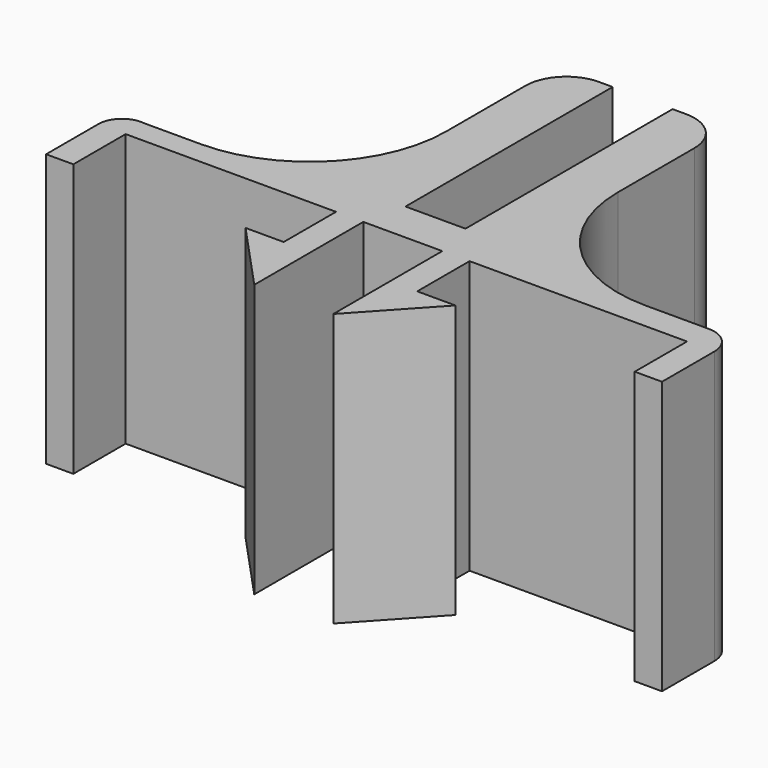
from build123d import *

# Parameters (mm, degrees)
F0_W     = 1
F0_H     = 2.4
F1_DEPTH = 10


# Not quite as in the source:
# - a feature names something its author has since deleted; it is built from what else it names


with BuildPart() as f1:
    # F0 (on Top) → F1 (new body)
    with BuildSketch(Plane.XY):
        with Locations((10.9311291858, -6.7)):
            Rectangle(F0_W, F0_H)
        with Locations((-10.6688708142, -6.7)):
            Rectangle(F0_W, F0_H)
        Polygon((-2.45, -8.5), (-2.45, -7.9), (-3.85, -7.9), (-1.45, -10.5), (-1.45, -8.5), align=None)
        with BuildLine():
            Line((-11.1688708142, -5.5), (-10.1688708142, -5.5))
            Line((-10.1688708142, -5.5), (-10.1688708142, -4.6410811281))
            ThreePointArc((-10.1688708142, -4.6410811281), (-10.8661281522, -4.8408828578), (-11.1688708142, -5.5))
        make_face()
        with BuildLine():
            Line((10.4311291858, -4.5), (10.4311291858, -5.5))
            Line((10.4311291858, -5.5), (11.4311291858, -5.5))
            ThreePointArc((11.4311291858, -5.5), (11.1382359669, -4.7928932188), (10.4311291858, -4.5))
        make_face()
        Polygon((-1.45, -5.5), (-2.45, -5.5), (-2.45, -7.9), (-2.45, -8.5), (-1.45, -8.5), align=None)
        Polygon((2.45, -5.5), (1.45, -5.5), (1.45, -8.5), (2.45, -8.5), (2.45, -7.9), align=None)
        with BuildLine():
            Line((-10.1688708142, -4.6410811281), (-10.1688708142, -5.5))
            Line((-10.1688708142, -5.5), (-2.45, -5.5))
            Line((-2.45, -5.5), (-1.45, -5.5))
            Line((-1.45, -5.5), (1.45, -5.5))
            Line((1.45, -5.5), (2.45, -5.5))
            Line((2.45, -5.5), (10.4311291858, -5.5))
            Line((10.4311291858, -5.5), (10.4311291858, -4.5))
            Line((10.4311291858, -4.5), (8.1, -4.5))
            ThreePointArc((8.1, -4.5), (4.5644660941, -3.0355339059), (3.1, 0.5))
            Line((3.1, 0.5), (3.1, 4))
            ThreePointArc((3.1, 4), (2.6606601718, 5.0606601718), (1.6, 5.5))
            Line((1.6, 5.5), (1.1, 5.5))
            Line((1.1, 5.5), (1.1, -4))
            Line((1.1, -4), (-1.1, -4))
            Line((-1.1, -4), (-1.1, 5.5))
            Line((-1.1, 5.5), (-1.6, 5.5))
            ThreePointArc((-1.6, 5.5), (-2.6606601718, 5.0606601718), (-3.1, 4))
            Line((-3.1, 4), (-3.1, 0.3589188719))
            ThreePointArc((-3.1, 0.3589188719), (-4.5644660941, -3.176615034), (-8.1, -4.6410811281))
            Line((-8.1, -4.6410811281), (-10.1688708142, -4.6410811281))
        make_face()
        Polygon((2.45, -8.5), (1.45, -8.5), (1.45, -10.5), (3.85, -7.9), (2.45, -7.9), align=None)
    extrude(amount=F1_DEPTH)


solid = f1.part
